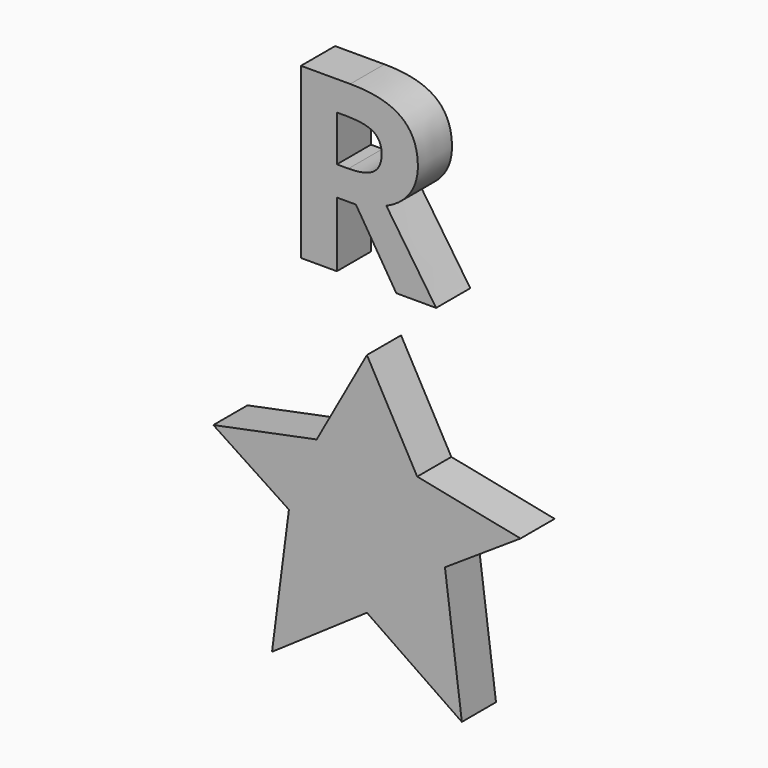
from build123d import *

# Parameters (mm, degrees)
F0_TEXT_SIZE = 35.2777777778
F1_DEPTH     = 6.35


# Not quite as in the source:
# - Text() gives the source's letters only with a copy of the font that has no kerning and outlines rounded to 1/6400 em; it was checked with that copy


with BuildPart() as f1:
    # F0 (on Front) → F1 (new body)
    with BuildSketch(Plane.XZ):
        with Locations((-12.9885624356, 33.5533187449)):
            Text('R', F0_TEXT_SIZE, font='Open Sans', font_style=FontStyle.BOLD, text_align=(TextAlign.LEFT, TextAlign.BOTTOM))
        Polygon((-11.6111217067, 0), (-14.1282569828, -19.4458774789), (0, -9.7337383777), (14.1282569828, -19.4458774789), (11.6111217067, 0), (22.86, 7.4276642559), (7.4823922478, 10.5345742777), (0, 24.0364264461), (-7.4823922478, 10.5345742777), (-22.86, 7.4276642559), align=None)
    extrude(amount=F1_DEPTH)


solid = f1.part
